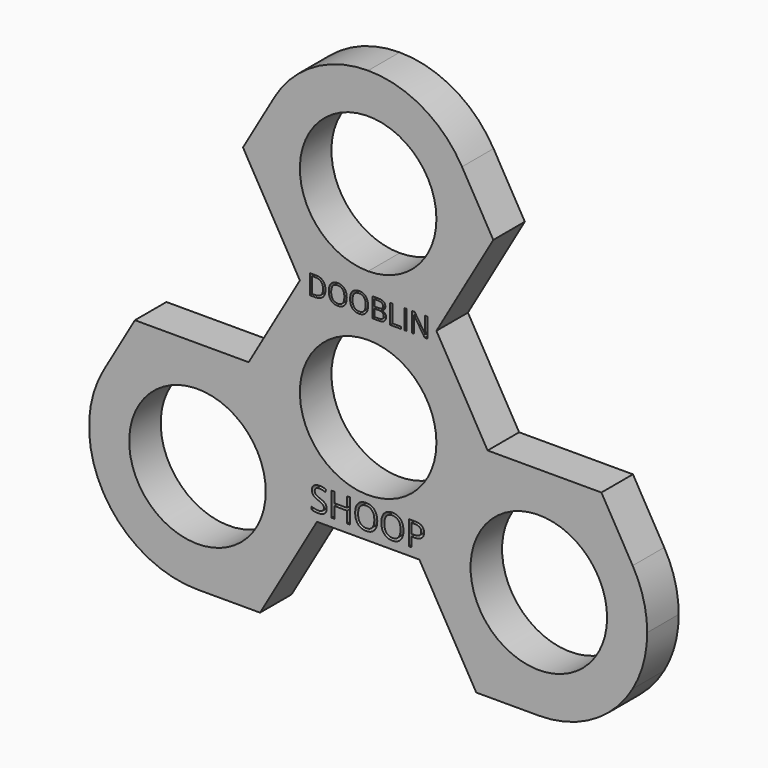
from build123d import *

# Parameters (mm, degrees)
F1_R         = 14.2875
F2_DEPTH     = 6.35
F3_TEXT_SIZE = 4.4097222222
F4_DEPTH     = 2.54
F6_DEPTH     = 25.4
F0_R         = 14.2875
F0_R_2       = 10.9982
F8_DEPTH     = 6.35
F9_TEXT_SIZE = 5.418546541
F10_DEPTH    = 2.54


# Not quite as in the source:
# - Text() gives the source's letters only with a copy of the font that has no kerning and outlines rounded to 1/6400 em; it was checked with that copy


with BuildPart() as f2:
    # F1 (on Front) → F2 (new body)
    with BuildSketch(Plane.XZ):
        Polygon((19.2474145991, 1.5875), (10.9985226281, 15.875), (20.1639581514, 31.75), (10.0819790757, 49.2125), (-10.0819790757, 49.2125), (-20.1639581514, 31.75), (-10.9985226281, 15.875), (-19.2474145991, 1.5875), (-37.5782856459, 1.5875), (-47.6602647216, -15.875), (-37.5782856459, -33.3375), (-17.4143274944, -33.3375), (-8.248891971, -17.4625), (8.248891971, -17.4625), (17.4143274944, -33.3375), (37.5782856459, -33.3375), (47.6602647216, -15.875), (37.5782856459, 1.5875), align=None)
        with Locations((-27.4963065702, -15.875)):
            Circle(F1_R, mode=Mode.SUBTRACT)
        with Locations((27.4963065702, -15.875)):
            Circle(F1_R, mode=Mode.SUBTRACT)
        Circle(F1_R, mode=Mode.SUBTRACT)
        with Locations((0, 31.75)):
            Circle(F1_R, mode=Mode.SUBTRACT)
    extrude(amount=F2_DEPTH)

    # F3 (on face) → F4 (cut)
    with BuildSketch(Plane.XZ.offset(6.35)):
        with Locations((-9.8247784904, 14.2875)):
            Text('DOOBLIN', F3_TEXT_SIZE, font='Open Sans', text_align=(TextAlign.LEFT, TextAlign.BOTTOM))
    extrude(amount=-F4_DEPTH, mode=Mode.SUBTRACT)

    # F5 (on face) → F6 (cut)
    with BuildSketch(Plane.XZ.offset(6.35)):
        with BuildLine():
            ThreePointArc((-15.1229685631, 40.4812500875), (-8.7312499563, 46.8729686388), (0, 49.2125))
            Line((0, 49.2125), (-10.0819790757, 49.2125))
            Line((-10.0819790757, 49.2125), (-15.1229685631, 40.4812500875))
        make_face()
        with BuildLine():
            ThreePointArc((0, 49.2125), (8.731250055, 46.8729685818), (15.1229686772, 40.4812498899))
            Line((15.1229686772, 40.4812498899), (10.0819790757, 49.2125))
            Line((10.0819790757, 49.2125), (0, 49.2125))
        make_face()
        with BuildLine():
            ThreePointArc((-42.6192755244, -24.60624941), (-44.9588065702, -15.8749996222), (-42.6192751466, -7.1437499356))
            Line((-42.6192751466, -7.1437499356), (-47.6602647216, -15.875))
            Line((-47.6602647216, -15.875), (-42.6192755244, -24.60624941))
        make_face()
        with BuildLine():
            ThreePointArc((-27.4963065702, -33.3375), (-36.2275568652, -30.9979684433), (-42.6192755244, -24.60624941))
            Line((-42.6192755244, -24.60624941), (-37.5782856459, -33.3375))
            Line((-37.5782856459, -33.3375), (-27.4963065702, -33.3375))
        make_face()
        with BuildLine():
            Line((37.5782856459, -33.3375), (42.6192787242, -24.6062438677))
            ThreePointArc((42.6192787242, -24.6062438677), (36.2275596363, -30.9979668433), (27.4963065702, -33.3375))
            Line((27.4963065702, -33.3375), (37.5782856459, -33.3375))
        make_face()
        with BuildLine():
            Line((47.6602647216, -15.875), (42.6192780426, -7.1437549517))
            ThreePointArc((42.6192780426, -7.1437549517), (44.3637870517, -11.3553751863), (44.9588065702, -15.875))
            ThreePointArc((44.9588065702, -15.875), (44.3637872281, -20.3946241552), (42.6192787242, -24.6062438677))
            Line((42.6192787242, -24.6062438677), (47.6602647216, -15.875))
        make_face()
    extrude(amount=-F6_DEPTH, mode=Mode.SUBTRACT)

    # F0 (on Front) → F8 (join)
    with BuildSketch(Plane.XZ):
        with Locations((-27.4963065702, -15.875)):
            Circle(F0_R)
        with Locations((-27.4963065702, -15.875)):
            Circle(F0_R_2, mode=Mode.SUBTRACT)
        with BuildLine():
            ThreePointArc((14.2875, 0), (10.1027881362, 10.1027881362), (0, 14.2875))
            ThreePointArc((0, 14.2875), (-10.1027881362, -10.1027881362), (14.2875, 0))
        make_face()
        with BuildLine():
            ThreePointArc((0, 10.9982), (7.7769018008, 7.7769018008), (10.9982, 0))
            ThreePointArc((10.9982, 0), (-7.7769018008, -7.7769018008), (0, 10.9982))
        make_face(mode=Mode.SUBTRACT)
        with Locations((27.4963065702, -15.875)):
            Circle(F0_R)
        with Locations((27.4963065702, -15.875)):
            Circle(F0_R_2, mode=Mode.SUBTRACT)
        with BuildLine():
            ThreePointArc((14.2875, 31.75), (-10.1027881362, 41.8527881362), (0, 17.4625))
            ThreePointArc((0, 17.4625), (10.1027881362, 21.6472118638), (14.2875, 31.75))
        make_face()
        with BuildLine():
            ThreePointArc((10.9982, 31.75), (7.7769018008, 23.9730981992), (0, 20.7518))
            ThreePointArc((0, 20.7518), (-7.7769018008, 39.5269018008), (10.9982, 31.75))
        make_face(mode=Mode.SUBTRACT)
    extrude(amount=F8_DEPTH)

    # F9 (on face) → F10 (cut)
    with BuildSketch(Plane.XZ.offset(6.35)):
        with Locations((-9.3920744974, -16.135128035)):
            Text('SHOOP', F9_TEXT_SIZE, font='Open Sans', text_align=(TextAlign.LEFT, TextAlign.BOTTOM))
    extrude(amount=-F10_DEPTH, mode=Mode.SUBTRACT)


solid = f2.part
